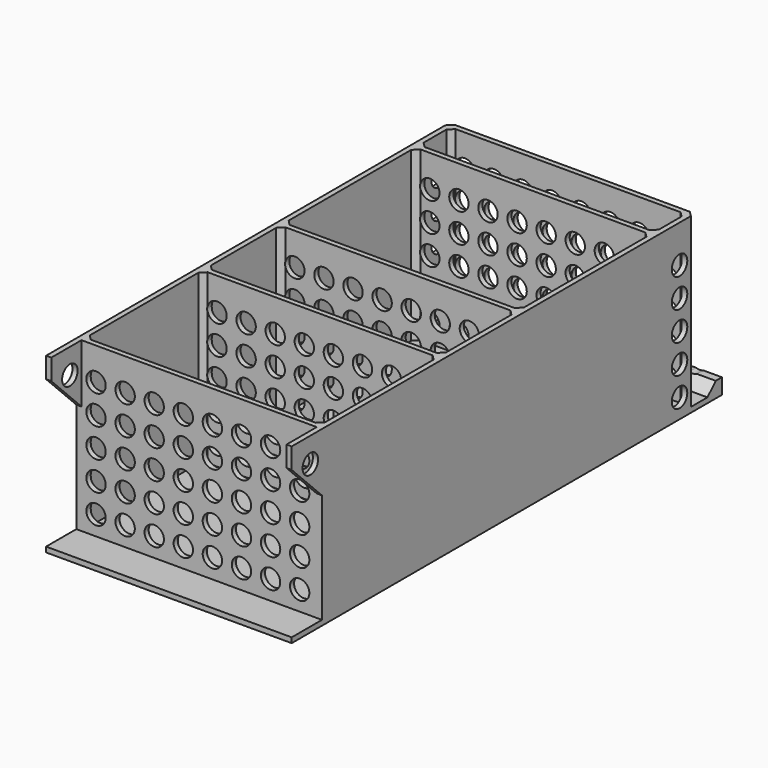
from build123d import *

# Parameters (mm, degrees)
F4_W           = 45.5
F4_H           = 63.25
F4_H_2         = 56.5
F4_H_3         = 35.625
F4_H_4         = 15
F4_H_5         = 6.2731353669
F4_W_2         = 95
F4_H_6         = 2
F5_DEPTH       = 2
F6_DEPTH       = 67
F7_DEPTH       = 6
F8_T4_DEPTH    = 95
F9_R           = 3.75
F10_DEPTH      = 187.8256165961
F10_DEPTH_BACK = 20.1763834039
F11_R          = 3.75
F12_DEPTH      = 47.501
F12_DEPTH_BACK = 47.501
F13_T4_DEPTH   = 70.1433659759
F13_S5_R       = 3.75
F13_T6_DEPTH   = 37
F13_S7_R       = 3.75
F13_T8_DEPTH   = 37
F13_S9_R       = 3.75
F13_T10_DEPTH  = 37
F13_S11_R      = 3.75
F13_T12_DEPTH  = 37
F13_S13_R      = 3.75
F13_T14_DEPTH  = 37
F13_T19_DEPTH  = 70.1433659759
F13_T24_DEPTH  = 70.1433659759
F13_S25_R      = 3.75
F13_T26_DEPTH  = 37
F13_S27_R      = 3.75
F13_T28_DEPTH  = 37
F13_S29_R      = 3.75
F13_T30_DEPTH  = 37
F13_S31_R      = 3.75
F13_T32_DEPTH  = 37
F13_S33_R      = 3.75
F13_T34_DEPTH  = 37
F13_S35_R      = 3.75
F13_T36_DEPTH  = 37
F13_S37_R      = 3.75
F13_T38_DEPTH  = 37
F13_S39_R      = 3.75
F13_T40_DEPTH  = 37
F13_S41_R      = 3.75
F13_T42_DEPTH  = 37
F13_S43_R      = 3.75
F13_T44_DEPTH  = 37
F13_T49_DEPTH  = 70.1433659759
F13_S50_R      = 3.75
F13_T51_DEPTH  = 37
F13_S52_R      = 3.75
F13_T53_DEPTH  = 37
F13_S54_R      = 3.75
F13_T55_DEPTH  = 37
F13_S56_R      = 3.75
F13_T57_DEPTH  = 37
F13_S58_R      = 3.75
F13_T59_DEPTH  = 37
F13_T64_DEPTH  = 70.1433659759
F13_S65_R      = 3.75
F13_T66_DEPTH  = 37
F13_S67_R      = 3.75
F13_T68_DEPTH  = 37
F13_S69_R      = 3.75
F13_T70_DEPTH  = 37
F13_S71_R      = 3.75
F13_T72_DEPTH  = 37
F13_S73_R      = 3.75
F13_T74_DEPTH  = 37
F13_T79_DEPTH  = 70.1433659759
F13_S80_R      = 3.75
F13_T81_DEPTH  = 37
F13_S82_R      = 3.75
F13_T83_DEPTH  = 37
F13_S84_R      = 3.75
F13_T85_DEPTH  = 37
F13_S86_R      = 3.75
F13_T87_DEPTH  = 37
F13_S88_R      = 3.75
F13_T89_DEPTH  = 37
F13_T94_DEPTH  = 70.1433659759
F13_T99_DEPTH  = 70.1433659759
F13_T104_DEPTH = 70.1433659759
F13_S105_R     = 3.75
F13_T106_DEPTH = 37
F13_S107_R     = 3.75
F13_T108_DEPTH = 37
F13_S109_R     = 3.75
F13_T110_DEPTH = 37
F13_S111_R     = 3.75
F13_T112_DEPTH = 37
F13_S113_R     = 3.75
F13_T114_DEPTH = 37
F13_T119_DEPTH = 70.1433659759
F13_T124_DEPTH = 70.1433659759
F13_S125_R     = 3.75
F13_T126_DEPTH = 37
F13_S127_R     = 3.75
F13_T128_DEPTH = 37
F13_S129_R     = 3.75
F13_T130_DEPTH = 37
F13_S131_R     = 3.75
F13_T132_DEPTH = 37
F13_S133_R     = 3.75
F13_T134_DEPTH = 37
F13_T139_DEPTH = 70.1433659759
F13_T144_DEPTH = 70.1433659759
F13_S145_R     = 3.75
F13_T146_DEPTH = 37
F13_S147_R     = 3.75
F13_T148_DEPTH = 37
F13_S149_R     = 3.75
F13_T150_DEPTH = 37
F13_S151_R     = 3.75
F13_T152_DEPTH = 37
F13_S153_R     = 3.75
F13_T154_DEPTH = 37
F13_T159_DEPTH = 70.1433659759
F13_T164_DEPTH = 70.1433659759
F13_T169_DEPTH = 70.1433659759
F13_S170_R     = 3.75
F13_T171_DEPTH = 37
F13_S172_R     = 3.75
F13_T173_DEPTH = 37
F13_S174_R     = 3.75
F13_T175_DEPTH = 37
F13_S176_R     = 3.75
F13_T177_DEPTH = 37
F13_S178_R     = 3.75
F13_T179_DEPTH = 37
F13_T181_DEPTH = 70.1433659759


# Not quite as in the source:
# - a fillet or chamfer that OpenCascade refuses, or shapes differently, is made with other operations: its cross-section is extruded or revolved along the edge and cut away or added
# - a feature names something its author has since deleted; it is built from what else it names


with BuildPart() as f5:
    # F4 (on Top) → F5 (new body)
    with BuildSketch(Plane.XY):
        Polygon((47.5, 174.8246165961), (0, 174.8246165961), (-47.5, 174.8246165961), (-47.5, -11.8235187708), (-47.5, -20.1753834039), (-45.5, -20.1753834039), (-45.5, -11.8235187708), (-45.5, -5.5503834039), (0, -5.5503834039), (45.5, -5.5503834039), (45.5, -11.8235187708), (45.5, -20.1753834039), (47.5, -20.1753834039), (47.5, -11.8235187708), align=None)
        Polygon((45.5, -3.5503834039), (0, -3.5503834039), (-45.5, -3.5503834039), (-45.5, 52.9496165961), (0, 52.9496165961), (45.5, 52.9496165961), align=None, mode=Mode.SUBTRACT)
        Polygon((45.5, 54.9496165961), (0, 54.9496165961), (-45.5, 54.9496165961), (-45.5, 90.5746165961), (-45.5, 92.5746165961), (-45.5, 155.8246165961), (-45.5, 157.8246165961), (-45.5, 172.8246165961), (0, 172.8246165961), (45.5, 172.8246165961), (45.5, 157.8246165961), (45.5, 155.8246165961), (45.5, 92.5746165961), (45.5, 90.5746165961), align=None, mode=Mode.SUBTRACT)
        with Locations((-22.75, 124.1996165961)):
            Rectangle(F4_W, F4_H)
        with Locations((22.75, 124.1996165961)):
            Rectangle(F4_W, F4_H)
        with Locations((22.75, 24.6996165961)):
            Rectangle(F4_W, F4_H_2)
        with Locations((-22.75, 24.6996165961)):
            Rectangle(F4_W, F4_H_2)
        with Locations((-22.75, 72.7621165961)):
            Rectangle(F4_W, F4_H_3)
        with Locations((22.75, 72.7621165961)):
            Rectangle(F4_W, F4_H_3)
        Polygon((-47.5, 174.8246165961), (0, 174.8246165961), (47.5, 174.8246165961), (47.5, 185.8246165961), (-47.5, 185.8246165961), align=None)
        Polygon((-45.5, -20.1753834039), (45.5, -20.1753834039), (45.5, -11.8235187708), (0, -11.8235187708), (-45.5, -11.8235187708), align=None)
        with Locations((-22.75, 165.3246165961)):
            Rectangle(F4_W, F4_H_4)
        with Locations((22.75, 165.3246165961)):
            Rectangle(F4_W, F4_H_4)
        with Locations((22.75, -8.6869510874)):
            Rectangle(F4_W, F4_H_5)
        with Locations((-22.75, -8.6869510874)):
            Rectangle(F4_W, F4_H_5)
        with Locations((0, 186.8246165961)):
            Rectangle(F4_W_2, F4_H_6)
        with Locations((-22.75, 156.8246165961)):
            Rectangle(F4_W, F4_H_6)
        with Locations((22.75, 156.8246165961)):
            Rectangle(F4_W, F4_H_6)
        with Locations((-22.75, 91.5746165961)):
            Rectangle(F4_W, F4_H_6)
        with Locations((22.75, 91.5746165961)):
            Rectangle(F4_W, F4_H_6)
    extrude(amount=F5_DEPTH)

    # F4 (on Top) → F6 (join)
    with BuildSketch(Plane.XY):
        Polygon((47.5, 174.8246165961), (0, 174.8246165961), (-47.5, 174.8246165961), (-47.5, -11.8235187708), (-47.5, -20.1753834039), (-45.5, -20.1753834039), (-45.5, -11.8235187708), (-45.5, -5.5503834039), (0, -5.5503834039), (45.5, -5.5503834039), (45.5, -11.8235187708), (45.5, -20.1753834039), (47.5, -20.1753834039), (47.5, -11.8235187708), align=None)
        Polygon((45.5, -3.5503834039), (0, -3.5503834039), (-45.5, -3.5503834039), (-45.5, 52.9496165961), (0, 52.9496165961), (45.5, 52.9496165961), align=None, mode=Mode.SUBTRACT)
        Polygon((45.5, 54.9496165961), (0, 54.9496165961), (-45.5, 54.9496165961), (-45.5, 90.5746165961), (-45.5, 92.5746165961), (-45.5, 155.8246165961), (-45.5, 157.8246165961), (-45.5, 172.8246165961), (0, 172.8246165961), (45.5, 172.8246165961), (45.5, 157.8246165961), (45.5, 155.8246165961), (45.5, 92.5746165961), (45.5, 90.5746165961), align=None, mode=Mode.SUBTRACT)
        with Locations((22.75, 156.8246165961)):
            Rectangle(F4_W, F4_H_6)
        with Locations((-22.75, 156.8246165961)):
            Rectangle(F4_W, F4_H_6)
        with Locations((22.75, 91.5746165961)):
            Rectangle(F4_W, F4_H_6)
        with Locations((-22.75, 91.5746165961)):
            Rectangle(F4_W, F4_H_6)
    extrude(amount=F6_DEPTH)

    # F4 (on Top) → F7 (join)
    with BuildSketch(Plane.XY):
        with Locations((0, 186.8246165961)):
            Rectangle(F4_W_2, F4_H_6)
    extrude(amount=F7_DEPTH)

    # F8: chamfer of 5 on 1 edges, made by hand


with BuildPart() as f8_tool2:
    # F8_s3 → F8_t4 (new body)
    with BuildSketch(Plane.YZ.offset(47.5)):
        Polygon((180.8246165961, 2), (185.8246165961, 7), (185.8246165961, 2), align=None)
    extrude(amount=-F8_T4_DEPTH)

    split(bisect_by=Plane.XY.offset(6), keep=Keep.BOTTOM)


with BuildPart() as f5_1:
    add(f5.part)

    # F8_t1: union F8_tool2
    add(f8_tool2.part)

    # F9 (on Front) → F10 (cut, two sides)
    with BuildSketch(Plane.XZ) as f10_sk:
        with Locations((-39.875, 9.5)):
            Circle(F9_R)
        with Locations((-39.875, 20.75)):
            Circle(F9_R)
        with Locations((-39.875, 32)):
            Circle(F9_R)
        with Locations((-39.875, 43.25)):
            Circle(F9_R)
        with Locations((-39.875, 54.5)):
            Circle(F9_R)
        with Locations((-28.625, 9.5)):
            Circle(F9_R)
        with Locations((-28.625, 20.75)):
            Circle(F9_R)
        with Locations((-28.625, 32)):
            Circle(F9_R)
        with Locations((-28.625, 43.25)):
            Circle(F9_R)
        with Locations((-28.625, 54.5)):
            Circle(F9_R)
        with Locations((-17.375, 9.5)):
            Circle(F9_R)
        with Locations((-17.375, 20.75)):
            Circle(F9_R)
        with Locations((-17.375, 32)):
            Circle(F9_R)
        with Locations((-17.375, 43.25)):
            Circle(F9_R)
        with Locations((-17.375, 54.5)):
            Circle(F9_R)
        with Locations((-6.125, 9.5)):
            Circle(F9_R)
        with Locations((-6.125, 20.75)):
            Circle(F9_R)
        with Locations((-6.125, 32)):
            Circle(F9_R)
        with Locations((-6.125, 43.25)):
            Circle(F9_R)
        with Locations((-6.125, 54.5)):
            Circle(F9_R)
        with Locations((5.125, 9.5)):
            Circle(F9_R)
        with Locations((5.125, 20.75)):
            Circle(F9_R)
        with Locations((5.125, 32)):
            Circle(F9_R)
        with Locations((5.125, 43.25)):
            Circle(F9_R)
        with Locations((5.125, 54.5)):
            Circle(F9_R)
        with Locations((16.375, 9.5)):
            Circle(F9_R)
        with Locations((16.375, 20.75)):
            Circle(F9_R)
        with Locations((16.375, 32)):
            Circle(F9_R)
        with Locations((16.375, 43.25)):
            Circle(F9_R)
        with Locations((16.375, 54.5)):
            Circle(F9_R)
        with Locations((27.625, 9.5)):
            Circle(F9_R)
        with Locations((27.625, 20.75)):
            Circle(F9_R)
        with Locations((27.625, 32)):
            Circle(F9_R)
        with Locations((27.625, 43.25)):
            Circle(F9_R)
        with Locations((27.625, 54.5)):
            Circle(F9_R)
        with Locations((38.875, 9.5)):
            Circle(F9_R)
        with Locations((38.875, 20.75)):
            Circle(F9_R)
        with Locations((38.875, 32)):
            Circle(F9_R)
        with Locations((38.875, 43.25)):
            Circle(F9_R)
        with Locations((38.875, 54.5)):
            Circle(F9_R)
    extrude(amount=-F10_DEPTH, mode=Mode.SUBTRACT)
    extrude(f10_sk.sketch, amount=F10_DEPTH_BACK, mode=Mode.SUBTRACT)

    # F11 (on Right) → F12 (cut, two sides)
    with BuildSketch(Plane.YZ) as f12_sk:
        Polygon((-5.5503834039, 2), (-5.5503834039, 44.375), (-20.1753834039, 59), (-20.1753834039, 2), align=None)
        with Locations((167.3246165961, 52.5)):
            Circle(F11_R)
        with Locations((167.3246165961, 41.25)):
            Circle(F11_R)
        with Locations((167.3246165961, 30)):
            Circle(F11_R)
        with Locations((167.3246165961, 18.75)):
            Circle(F11_R)
        with Locations((167.3246165961, 7.5)):
            Circle(F11_R)
        with Locations((-11.1753834039, 57.375)):
            Circle(F11_R)
    extrude(amount=-F12_DEPTH, mode=Mode.SUBTRACT)
    extrude(f12_sk.sketch, amount=F12_DEPTH_BACK, mode=Mode.SUBTRACT)

    # F13: chamfer of 2 on 18 edges, made by hand


with BuildPart() as f13_tool2:
    # F13_s3 → F13_t4 (new body)
    with BuildSketch(Plane.XY.offset(-3.1433659759)):
        Polygon((-45.5, -1.5503834039), (-43.5, -3.5503834039), (-45.5, -3.5503834039), align=None)
    extrude(amount=F13_T4_DEPTH)

    # F13_s5 → F13_t6 (cut, symmetric)
    with BuildSketch(Plane.XZ.offset(2.6)):
        with Locations((-39.875, 9.5)):
            Circle(F13_S5_R)
    extrude(amount=F13_T6_DEPTH, both=True, mode=Mode.SUBTRACT)

    # F13_s7 → F13_t8 (cut, symmetric)
    with BuildSketch(Plane.XZ.offset(2.6)):
        with Locations((-39.875, 20.75)):
            Circle(F13_S7_R)
    extrude(amount=F13_T8_DEPTH, both=True, mode=Mode.SUBTRACT)

    # F13_s9 → F13_t10 (cut, symmetric)
    with BuildSketch(Plane.XZ.offset(2.6)):
        with Locations((-39.875, 32)):
            Circle(F13_S9_R)
    extrude(amount=F13_T10_DEPTH, both=True, mode=Mode.SUBTRACT)

    # F13_s11 → F13_t12 (cut, symmetric)
    with BuildSketch(Plane.XZ.offset(2.6)):
        with Locations((-39.875, 43.25)):
            Circle(F13_S11_R)
    extrude(amount=F13_T12_DEPTH, both=True, mode=Mode.SUBTRACT)

    # F13_s13 → F13_t14 (cut, symmetric)
    with BuildSketch(Plane.XZ.offset(2.6)):
        with Locations((-39.875, 54.5)):
            Circle(F13_S13_R)
    extrude(amount=F13_T14_DEPTH, both=True, mode=Mode.SUBTRACT)

    split(bisect_by=Plane.XY, keep=Keep.TOP)


with BuildPart() as f5_2:
    add(f5_1.part)

    # F13_t1: union F13_tool2
    add(f13_tool2.part)


with BuildPart() as f13_tool17:
    # F13_s18 → F13_t19 (new body)
    with BuildSketch(Plane.XY.offset(-3.1433659759)):
        Polygon((43.5, -3.5503834039), (45.5, -1.5503834039), (45.5, -3.5503834039), align=None)
    extrude(amount=F13_T19_DEPTH)

    split(bisect_by=Plane.XY, keep=Keep.TOP)


with BuildPart() as f5_3:
    add(f5_2.part)

    # F13_t16: union F13_tool17
    add(f13_tool17.part)


with BuildPart() as f13_tool22:
    # F13_s23 → F13_t24 (new body)
    with BuildSketch(Plane.XY.offset(-3.1433659759)):
        Polygon((-43.5, 172.8246165961), (-45.5, 170.8246165961), (-45.5, 172.8246165961), align=None)
    extrude(amount=F13_T24_DEPTH)

    # F13_s25 → F13_t26 (cut, symmetric)
    with BuildSketch(Plane.XZ.offset(-171.8)):
        with Locations((-39.875, 9.5)):
            Circle(F13_S25_R)
    extrude(amount=F13_T26_DEPTH, both=True, mode=Mode.SUBTRACT)

    # F13_s27 → F13_t28 (cut, symmetric)
    with BuildSketch(Plane.YZ.offset(-44.5)):
        with Locations((167.3246165961, 7.5)):
            Circle(F13_S27_R)
    extrude(amount=F13_T28_DEPTH, both=True, mode=Mode.SUBTRACT)

    # F13_s29 → F13_t30 (cut, symmetric)
    with BuildSketch(Plane.YZ.offset(-44.5)):
        with Locations((167.3246165961, 18.75)):
            Circle(F13_S29_R)
    extrude(amount=F13_T30_DEPTH, both=True, mode=Mode.SUBTRACT)

    # F13_s31 → F13_t32 (cut, symmetric)
    with BuildSketch(Plane.YZ.offset(-44.5)):
        with Locations((167.3246165961, 30)):
            Circle(F13_S31_R)
    extrude(amount=F13_T32_DEPTH, both=True, mode=Mode.SUBTRACT)

    # F13_s33 → F13_t34 (cut, symmetric)
    with BuildSketch(Plane.YZ.offset(-44.5)):
        with Locations((167.3246165961, 41.25)):
            Circle(F13_S33_R)
    extrude(amount=F13_T34_DEPTH, both=True, mode=Mode.SUBTRACT)

    # F13_s35 → F13_t36 (cut, symmetric)
    with BuildSketch(Plane.YZ.offset(-44.5)):
        with Locations((167.3246165961, 52.5)):
            Circle(F13_S35_R)
    extrude(amount=F13_T36_DEPTH, both=True, mode=Mode.SUBTRACT)

    # F13_s37 → F13_t38 (cut, symmetric)
    with BuildSketch(Plane.XZ.offset(-171.8)):
        with Locations((-39.875, 20.75)):
            Circle(F13_S37_R)
    extrude(amount=F13_T38_DEPTH, both=True, mode=Mode.SUBTRACT)

    # F13_s39 → F13_t40 (cut, symmetric)
    with BuildSketch(Plane.XZ.offset(-171.8)):
        with Locations((-39.875, 32)):
            Circle(F13_S39_R)
    extrude(amount=F13_T40_DEPTH, both=True, mode=Mode.SUBTRACT)

    # F13_s41 → F13_t42 (cut, symmetric)
    with BuildSketch(Plane.XZ.offset(-171.8)):
        with Locations((-39.875, 43.25)):
            Circle(F13_S41_R)
    extrude(amount=F13_T42_DEPTH, both=True, mode=Mode.SUBTRACT)

    # F13_s43 → F13_t44 (cut, symmetric)
    with BuildSketch(Plane.XZ.offset(-171.8)):
        with Locations((-39.875, 54.5)):
            Circle(F13_S43_R)
    extrude(amount=F13_T44_DEPTH, both=True, mode=Mode.SUBTRACT)

    split(bisect_by=Plane.XY, keep=Keep.TOP)


with BuildPart() as f5_4:
    add(f5_3.part)

    # F13_t21: union F13_tool22
    add(f13_tool22.part)


with BuildPart() as f13_tool47:
    # F13_s48 → F13_t49 (new body)
    with BuildSketch(Plane.XY.offset(-3.1433659759)):
        Polygon((43.5, 172.8246165961), (45.5, 170.8246165961), (45.5, 172.8246165961), align=None)
    extrude(amount=F13_T49_DEPTH)

    # F13_s50 → F13_t51 (cut, symmetric)
    with BuildSketch(Plane.YZ.offset(44.5)):
        with Locations((167.3246165961, 7.5)):
            Circle(F13_S50_R)
    extrude(amount=F13_T51_DEPTH, both=True, mode=Mode.SUBTRACT)

    # F13_s52 → F13_t53 (cut, symmetric)
    with BuildSketch(Plane.YZ.offset(44.5)):
        with Locations((167.3246165961, 18.75)):
            Circle(F13_S52_R)
    extrude(amount=F13_T53_DEPTH, both=True, mode=Mode.SUBTRACT)

    # F13_s54 → F13_t55 (cut, symmetric)
    with BuildSketch(Plane.YZ.offset(44.5)):
        with Locations((167.3246165961, 30)):
            Circle(F13_S54_R)
    extrude(amount=F13_T55_DEPTH, both=True, mode=Mode.SUBTRACT)

    # F13_s56 → F13_t57 (cut, symmetric)
    with BuildSketch(Plane.YZ.offset(44.5)):
        with Locations((167.3246165961, 41.25)):
            Circle(F13_S56_R)
    extrude(amount=F13_T57_DEPTH, both=True, mode=Mode.SUBTRACT)

    # F13_s58 → F13_t59 (cut, symmetric)
    with BuildSketch(Plane.YZ.offset(44.5)):
        with Locations((167.3246165961, 52.5)):
            Circle(F13_S58_R)
    extrude(amount=F13_T59_DEPTH, both=True, mode=Mode.SUBTRACT)

    split(bisect_by=Plane.XY, keep=Keep.TOP)


with BuildPart() as f5_5:
    add(f5_4.part)

    # F13_t46: union F13_tool47
    add(f13_tool47.part)


with BuildPart() as f13_tool62:
    # F13_s63 → F13_t64 (new body)
    with BuildSketch(Plane.XY.offset(-3.1433659759)):
        Polygon((-43.5, 52.9496165961), (-45.5, 50.9496165961), (-45.5, 52.9496165961), align=None)
    extrude(amount=F13_T64_DEPTH)

    # F13_s65 → F13_t66 (cut, symmetric)
    with BuildSketch(Plane.XZ.offset(-51.9)):
        with Locations((-39.875, 9.5)):
            Circle(F13_S65_R)
    extrude(amount=F13_T66_DEPTH, both=True, mode=Mode.SUBTRACT)

    # F13_s67 → F13_t68 (cut, symmetric)
    with BuildSketch(Plane.XZ.offset(-51.9)):
        with Locations((-39.875, 20.75)):
            Circle(F13_S67_R)
    extrude(amount=F13_T68_DEPTH, both=True, mode=Mode.SUBTRACT)

    # F13_s69 → F13_t70 (cut, symmetric)
    with BuildSketch(Plane.XZ.offset(-51.9)):
        with Locations((-39.875, 32)):
            Circle(F13_S69_R)
    extrude(amount=F13_T70_DEPTH, both=True, mode=Mode.SUBTRACT)

    # F13_s71 → F13_t72 (cut, symmetric)
    with BuildSketch(Plane.XZ.offset(-51.9)):
        with Locations((-39.875, 43.25)):
            Circle(F13_S71_R)
    extrude(amount=F13_T72_DEPTH, both=True, mode=Mode.SUBTRACT)

    # F13_s73 → F13_t74 (cut, symmetric)
    with BuildSketch(Plane.XZ.offset(-51.9)):
        with Locations((-39.875, 54.5)):
            Circle(F13_S73_R)
    extrude(amount=F13_T74_DEPTH, both=True, mode=Mode.SUBTRACT)

    split(bisect_by=Plane.XY, keep=Keep.TOP)


with BuildPart() as f5_6:
    add(f5_5.part)

    # F13_t61: union F13_tool62
    add(f13_tool62.part)


with BuildPart() as f13_tool77:
    # F13_s78 → F13_t79 (new body)
    with BuildSketch(Plane.XY.offset(-3.1433659759)):
        Polygon((-45.5, 56.9496165961), (-43.5, 54.9496165961), (-45.5, 54.9496165961), align=None)
    extrude(amount=F13_T79_DEPTH)

    # F13_s80 → F13_t81 (cut, symmetric)
    with BuildSketch(Plane.XZ.offset(-55.9)):
        with Locations((-39.875, 9.5)):
            Circle(F13_S80_R)
    extrude(amount=F13_T81_DEPTH, both=True, mode=Mode.SUBTRACT)

    # F13_s82 → F13_t83 (cut, symmetric)
    with BuildSketch(Plane.XZ.offset(-55.9)):
        with Locations((-39.875, 20.75)):
            Circle(F13_S82_R)
    extrude(amount=F13_T83_DEPTH, both=True, mode=Mode.SUBTRACT)

    # F13_s84 → F13_t85 (cut, symmetric)
    with BuildSketch(Plane.XZ.offset(-55.9)):
        with Locations((-39.875, 32)):
            Circle(F13_S84_R)
    extrude(amount=F13_T85_DEPTH, both=True, mode=Mode.SUBTRACT)

    # F13_s86 → F13_t87 (cut, symmetric)
    with BuildSketch(Plane.XZ.offset(-55.9)):
        with Locations((-39.875, 43.25)):
            Circle(F13_S86_R)
    extrude(amount=F13_T87_DEPTH, both=True, mode=Mode.SUBTRACT)

    # F13_s88 → F13_t89 (cut, symmetric)
    with BuildSketch(Plane.XZ.offset(-55.9)):
        with Locations((-39.875, 54.5)):
            Circle(F13_S88_R)
    extrude(amount=F13_T89_DEPTH, both=True, mode=Mode.SUBTRACT)

    split(bisect_by=Plane.XY, keep=Keep.TOP)


with BuildPart() as f5_7:
    add(f5_6.part)

    # F13_t76: union F13_tool77
    add(f13_tool77.part)


with BuildPart() as f13_tool92:
    # F13_s93 → F13_t94 (new body)
    with BuildSketch(Plane.XY.offset(-3.1433659759)):
        Polygon((43.5, 52.9496165961), (45.5, 50.9496165961), (45.5, 52.9496165961), align=None)
    extrude(amount=F13_T94_DEPTH)

    split(bisect_by=Plane.XY, keep=Keep.TOP)


with BuildPart() as f5_8:
    add(f5_7.part)

    # F13_t91: union F13_tool92
    add(f13_tool92.part)


with BuildPart() as f13_tool97:
    # F13_s98 → F13_t99 (new body)
    with BuildSketch(Plane.XY.offset(-3.1433659759)):
        Polygon((43.5, 54.9496165961), (45.5, 56.9496165961), (45.5, 54.9496165961), align=None)
    extrude(amount=F13_T99_DEPTH)

    split(bisect_by=Plane.XY, keep=Keep.TOP)


with BuildPart() as f5_9:
    add(f5_8.part)

    # F13_t96: union F13_tool97
    add(f13_tool97.part)


with BuildPart() as f13_tool102:
    # F13_s103 → F13_t104 (new body)
    with BuildSketch(Plane.XY.offset(-3.1433659759)):
        Polygon((-45.5, 159.8246165961), (-43.5, 157.8246165961), (-45.5, 157.8246165961), align=None)
    extrude(amount=F13_T104_DEPTH)

    # F13_s105 → F13_t106 (cut, symmetric)
    with BuildSketch(Plane.XZ.offset(-158.8)):
        with Locations((-39.875, 9.5)):
            Circle(F13_S105_R)
    extrude(amount=F13_T106_DEPTH, both=True, mode=Mode.SUBTRACT)

    # F13_s107 → F13_t108 (cut, symmetric)
    with BuildSketch(Plane.XZ.offset(-158.8)):
        with Locations((-39.875, 20.75)):
            Circle(F13_S107_R)
    extrude(amount=F13_T108_DEPTH, both=True, mode=Mode.SUBTRACT)

    # F13_s109 → F13_t110 (cut, symmetric)
    with BuildSketch(Plane.XZ.offset(-158.8)):
        with Locations((-39.875, 32)):
            Circle(F13_S109_R)
    extrude(amount=F13_T110_DEPTH, both=True, mode=Mode.SUBTRACT)

    # F13_s111 → F13_t112 (cut, symmetric)
    with BuildSketch(Plane.XZ.offset(-158.8)):
        with Locations((-39.875, 43.25)):
            Circle(F13_S111_R)
    extrude(amount=F13_T112_DEPTH, both=True, mode=Mode.SUBTRACT)

    # F13_s113 → F13_t114 (cut, symmetric)
    with BuildSketch(Plane.XZ.offset(-158.8)):
        with Locations((-39.875, 54.5)):
            Circle(F13_S113_R)
    extrude(amount=F13_T114_DEPTH, both=True, mode=Mode.SUBTRACT)

    split(bisect_by=Plane.XY, keep=Keep.TOP)


with BuildPart() as f5_10:
    add(f5_9.part)

    # F13_t101: union F13_tool102
    add(f13_tool102.part)


with BuildPart() as f13_tool117:
    # F13_s118 → F13_t119 (new body)
    with BuildSketch(Plane.XY.offset(-3.1433659759)):
        Polygon((43.5, 157.8246165961), (45.5, 159.8246165961), (45.5, 157.8246165961), align=None)
    extrude(amount=F13_T119_DEPTH)

    split(bisect_by=Plane.XY, keep=Keep.TOP)


with BuildPart() as f5_11:
    add(f5_10.part)

    # F13_t116: union F13_tool117
    add(f13_tool117.part)


with BuildPart() as f13_tool122:
    # F13_s123 → F13_t124 (new body)
    with BuildSketch(Plane.XY.offset(-3.1433659759)):
        Polygon((-43.5, 155.8246165961), (-45.5, 153.8246165961), (-45.5, 155.8246165961), align=None)
    extrude(amount=F13_T124_DEPTH)

    # F13_s125 → F13_t126 (cut, symmetric)
    with BuildSketch(Plane.XZ.offset(-154.8)):
        with Locations((-39.875, 9.5)):
            Circle(F13_S125_R)
    extrude(amount=F13_T126_DEPTH, both=True, mode=Mode.SUBTRACT)

    # F13_s127 → F13_t128 (cut, symmetric)
    with BuildSketch(Plane.XZ.offset(-154.8)):
        with Locations((-39.875, 20.75)):
            Circle(F13_S127_R)
    extrude(amount=F13_T128_DEPTH, both=True, mode=Mode.SUBTRACT)

    # F13_s129 → F13_t130 (cut, symmetric)
    with BuildSketch(Plane.XZ.offset(-154.8)):
        with Locations((-39.875, 32)):
            Circle(F13_S129_R)
    extrude(amount=F13_T130_DEPTH, both=True, mode=Mode.SUBTRACT)

    # F13_s131 → F13_t132 (cut, symmetric)
    with BuildSketch(Plane.XZ.offset(-154.8)):
        with Locations((-39.875, 43.25)):
            Circle(F13_S131_R)
    extrude(amount=F13_T132_DEPTH, both=True, mode=Mode.SUBTRACT)

    # F13_s133 → F13_t134 (cut, symmetric)
    with BuildSketch(Plane.XZ.offset(-154.8)):
        with Locations((-39.875, 54.5)):
            Circle(F13_S133_R)
    extrude(amount=F13_T134_DEPTH, both=True, mode=Mode.SUBTRACT)

    split(bisect_by=Plane.XY, keep=Keep.TOP)


with BuildPart() as f5_12:
    add(f5_11.part)

    # F13_t121: union F13_tool122
    add(f13_tool122.part)


with BuildPart() as f13_tool137:
    # F13_s138 → F13_t139 (new body)
    with BuildSketch(Plane.XY.offset(-3.1433659759)):
        Polygon((43.5, 155.8246165961), (45.5, 153.8246165961), (45.5, 155.8246165961), align=None)
    extrude(amount=F13_T139_DEPTH)

    split(bisect_by=Plane.XY, keep=Keep.TOP)


with BuildPart() as f5_13:
    add(f5_12.part)

    # F13_t136: union F13_tool137
    add(f13_tool137.part)


with BuildPart() as f13_tool142:
    # F13_s143 → F13_t144 (new body)
    with BuildSketch(Plane.XY.offset(-3.1433659759)):
        Polygon((-43.5, 90.5746165961), (-45.5, 88.5746165961), (-45.5, 90.5746165961), align=None)
    extrude(amount=F13_T144_DEPTH)

    # F13_s145 → F13_t146 (cut, symmetric)
    with BuildSketch(Plane.XZ.offset(-89.6)):
        with Locations((-39.875, 9.5)):
            Circle(F13_S145_R)
    extrude(amount=F13_T146_DEPTH, both=True, mode=Mode.SUBTRACT)

    # F13_s147 → F13_t148 (cut, symmetric)
    with BuildSketch(Plane.XZ.offset(-89.6)):
        with Locations((-39.875, 20.75)):
            Circle(F13_S147_R)
    extrude(amount=F13_T148_DEPTH, both=True, mode=Mode.SUBTRACT)

    # F13_s149 → F13_t150 (cut, symmetric)
    with BuildSketch(Plane.XZ.offset(-89.6)):
        with Locations((-39.875, 32)):
            Circle(F13_S149_R)
    extrude(amount=F13_T150_DEPTH, both=True, mode=Mode.SUBTRACT)

    # F13_s151 → F13_t152 (cut, symmetric)
    with BuildSketch(Plane.XZ.offset(-89.6)):
        with Locations((-39.875, 43.25)):
            Circle(F13_S151_R)
    extrude(amount=F13_T152_DEPTH, both=True, mode=Mode.SUBTRACT)

    # F13_s153 → F13_t154 (cut, symmetric)
    with BuildSketch(Plane.XZ.offset(-89.6)):
        with Locations((-39.875, 54.5)):
            Circle(F13_S153_R)
    extrude(amount=F13_T154_DEPTH, both=True, mode=Mode.SUBTRACT)

    split(bisect_by=Plane.XY, keep=Keep.TOP)


with BuildPart() as f5_14:
    add(f5_13.part)

    # F13_t141: union F13_tool142
    add(f13_tool142.part)


with BuildPart() as f13_tool157:
    # F13_s158 → F13_t159 (new body)
    with BuildSketch(Plane.XY.offset(-3.1433659759)):
        Polygon((43.5, 90.5746165961), (45.5, 88.5746165961), (45.5, 90.5746165961), align=None)
    extrude(amount=F13_T159_DEPTH)

    split(bisect_by=Plane.XY, keep=Keep.TOP)


with BuildPart() as f5_15:
    add(f5_14.part)

    # F13_t156: union F13_tool157
    add(f13_tool157.part)


with BuildPart() as f13_tool162:
    # F13_s163 → F13_t164 (new body)
    with BuildSketch(Plane.XY.offset(-3.1433659759)):
        Polygon((43.5, 92.5746165961), (45.5, 94.5746165961), (45.5, 92.5746165961), align=None)
    extrude(amount=F13_T164_DEPTH)

    split(bisect_by=Plane.XY, keep=Keep.TOP)


with BuildPart() as f5_16:
    add(f5_15.part)

    # F13_t161: union F13_tool162
    add(f13_tool162.part)


with BuildPart() as f13_tool167:
    # F13_s168 → F13_t169 (new body)
    with BuildSketch(Plane.XY.offset(-3.1433659759)):
        Polygon((-45.5, 94.5746165961), (-43.5, 92.5746165961), (-45.5, 92.5746165961), align=None)
    extrude(amount=F13_T169_DEPTH)

    # F13_s170 → F13_t171 (cut, symmetric)
    with BuildSketch(Plane.XZ.offset(-93.6)):
        with Locations((-39.875, 9.5)):
            Circle(F13_S170_R)
    extrude(amount=F13_T171_DEPTH, both=True, mode=Mode.SUBTRACT)

    # F13_s172 → F13_t173 (cut, symmetric)
    with BuildSketch(Plane.XZ.offset(-93.6)):
        with Locations((-39.875, 20.75)):
            Circle(F13_S172_R)
    extrude(amount=F13_T173_DEPTH, both=True, mode=Mode.SUBTRACT)

    # F13_s174 → F13_t175 (cut, symmetric)
    with BuildSketch(Plane.XZ.offset(-93.6)):
        with Locations((-39.875, 32)):
            Circle(F13_S174_R)
    extrude(amount=F13_T175_DEPTH, both=True, mode=Mode.SUBTRACT)

    # F13_s176 → F13_t177 (cut, symmetric)
    with BuildSketch(Plane.XZ.offset(-93.6)):
        with Locations((-39.875, 43.25)):
            Circle(F13_S176_R)
    extrude(amount=F13_T177_DEPTH, both=True, mode=Mode.SUBTRACT)

    # F13_s178 → F13_t179 (cut, symmetric)
    with BuildSketch(Plane.XZ.offset(-93.6)):
        with Locations((-39.875, 54.5)):
            Circle(F13_S178_R)
    extrude(amount=F13_T179_DEPTH, both=True, mode=Mode.SUBTRACT)

    split(bisect_by=Plane.XY, keep=Keep.TOP)


with BuildPart() as f5_17:
    add(f5_16.part)

    # F13_t166: union F13_tool167
    add(f13_tool167.part)

    # F13_s182 → F13_t181 (cut)
    with BuildSketch(Plane.XY.offset(2)):
        Polygon((-45.5, 174.8246165961), (-47.5, 172.8246165961), (-47.5, 174.8246165961), align=None)
        Polygon((45.5, 174.8246165961), (47.5, 172.8246165961), (47.5, 174.8246165961), align=None)
    extrude(amount=F13_T181_DEPTH, mode=Mode.SUBTRACT)


solid = f5_17.part
